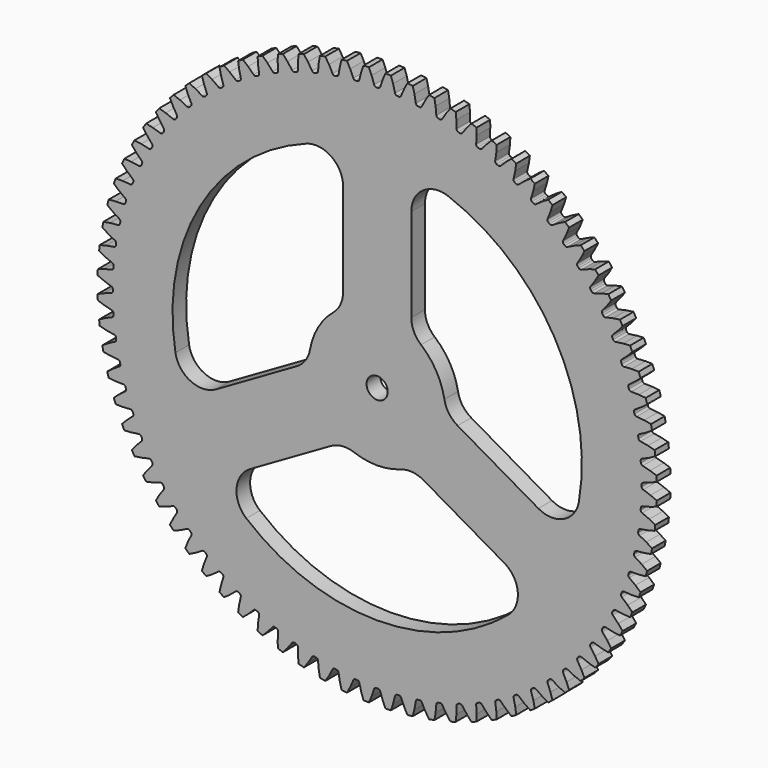
from build123d import *

# Parameters (mm, degrees)
F0_R     = 3.1
F1_DEPTH = 5


# Not quite as in the source:
# - ends of sketch curves that miss each other by under 0.0002 mm in the source are joined


with BuildPart() as f1:
    # F0 (on Front) → F1 (new body)
    with BuildSketch(Plane.XZ):
        with BuildLine():
            ThreePointArc((-66.025163696, 41.5067142777), (-65.8531282029, 41.1183062198), (-65.9498350759, 40.7046580468))
            ThreePointArc((-65.9498350759, 40.7046580468), (-66.0796127847, 40.4936386884), (-66.2087146573, 40.2822057915))
            ThreePointArc((-66.2087146573, 40.2822057915), (-66.5333738388, 40.0082469182), (-66.9575511036, 39.9851986244))
            Line((-66.9575511036, 39.9851986244), (-69.17445, 40.481426))
            Line((-69.17445, 40.481426), (-71.152959, 40.758514))
            ThreePointArc((-71.152959, 40.758514), (-71.5446727033, 40.0669415825), (-71.929665068, 39.3716050372))
            Line((-71.929665068, 39.3716050372), (-70.65964, 37.829428))
            Line((-70.65964, 37.829428), (-69.07821, 36.198488))
            ThreePointArc((-69.07821, 36.198488), (-68.8762309064, 35.8247752552), (-68.9401849616, 35.4048149803))
            ThreePointArc((-68.9401849616, 35.4048149803), (-69.0530056484, 35.1842636831), (-69.1651209082, 34.9633529536))
            ThreePointArc((-69.1651209082, 34.9633529536), (-69.467284766, 34.6647666816), (-69.888344948, 34.6085082698))
            Line((-69.888344948, 34.6085082698), (-72.137344, 34.92927))
            Line((-72.137344, 34.92927), (-74.131494, 35.050273))
            ThreePointArc((-74.131494, 35.050273), (-74.4677401642, 34.3300986722), (-74.7969903852, 33.6066991731))
            Line((-74.7969903852, 33.6066991731), (-73.409883, 32.168921))
            Line((-73.409883, 32.168921), (-71.705366, 30.667087))
            ThreePointArc((-71.705366, 30.667087), (-71.4746875004, 30.3103731451), (-71.5054948793, 29.8866889496))
            ThreePointArc((-71.5054948793, 29.8866889496), (-71.6006637701, 29.6579660072), (-71.695100899, 29.4289399585))
            ThreePointArc((-71.695100899, 29.4289399585), (-71.9729063671, 29.1075663054), (-72.3882550299, 29.0184457338))
            Line((-72.3882550299, 29.0184457338), (-74.655488, 29.161764))
            Line((-74.655488, 29.161764), (-76.652984, 29.125934))
            ThreePointArc((-76.652984, 29.125934), (-76.9316895099, 28.3815987773), (-77.203167309, 27.6345971106))
            Line((-77.203167309, 27.6345971106), (-75.707529, 26.310081))
            Line((-75.707529, 26.310081), (-73.890434, 24.946612))
            ThreePointArc((-73.890434, 24.946612), (-73.6324790283, 24.6090973171), (-73.6299495486, 24.1843018517))
            ThreePointArc((-73.6299495486, 24.1843018517), (-73.7068799327, 23.9488173109), (-73.7830567374, 23.7130879156))
            ThreePointArc((-73.7830567374, 23.7130879156), (-74.0347910448, 23.3709082224), (-74.4418670003, 23.2494739916))
            Line((-74.4418670003, 23.2494739916), (-76.713356, 23.214466))
            Line((-76.713356, 23.214466), (-78.701883, 23.022025))
            ThreePointArc((-78.701883, 23.022025), (-78.9213293367, 22.2581170751), (-79.1333612396, 21.4921180651))
            Line((-79.1333612396, 21.4921180651), (-77.538413, 20.289032))
            Line((-77.538413, 20.289032), (-75.619943, 19.072333))
            ThreePointArc((-75.619943, 19.072333), (-75.3363026573, 18.7560970153), (-75.300452163, 18.3328100397))
            ThreePointArc((-75.300452163, 18.3328100397), (-75.3586689009, 18.092015407), (-75.4161157564, 17.8510359423))
            ThreePointArc((-75.4161157564, 17.8510359423), (-75.640226983, 17.4901601634), (-76.0365209903, 17.3371617849))
            Line((-76.0365209903, 17.3371617849), (-78.29826, 17.124043))
            Line((-78.29826, 17.124043), (-80.265558, 16.776177))
            ThreePointArc((-80.265558, 16.776177), (-80.4243929961, 15.99740639), (-80.5756716705, 15.2171329378))
            Line((-80.5756716705, 15.2171329378), (-78.891247, 14.142894))
            Line((-78.891247, 14.142894), (-76.88323, 13.080467))
            ThreePointArc((-76.88323, 13.080467), (-76.5756525366, 12.7874601089), (-76.5067014576, 12.368291074))
            ThreePointArc((-76.5067014576, 12.368291074), (-76.5458464162, 12.123670914), (-76.5842091605, 11.8789270249))
            ThreePointArc((-76.5842091605, 11.8789270249), (-76.7793160154, 11.5015804485), (-77.1623840176, 11.3179611415))
            Line((-77.1623840176, 11.3179611415), (-79.400429, 10.928045))
            Line((-79.400429, 10.928045), (-81.33437, 10.426899))
            ThreePointArc((-81.33437, 10.426899), (-81.431613449, 9.6380667714), (-81.5212062801, 8.8483290304))
            Line((-81.5212062801, 8.8483290304), (-79.757691, 7.90956))
            Line((-79.757691, 7.90956), (-77.672506, 7.007956))
            ThreePointArc((-77.672506, 7.007956), (-77.3428878657, 6.7399838602), (-77.2412619261, 6.3275169939))
            ThreePointArc((-77.2412619261, 6.3275169939), (-77.2610933521, 6.0805800746), (-77.2801354317, 5.8335810326))
            ThreePointArc((-77.2801354317, 5.8335810326), (-77.4450345987, 5.4420896099), (-77.8125149825, 5.2289809145))
            Line((-77.8125149825, 5.2289809145), (-80.013069, 4.664671))
            Line((-80.013069, 4.664671), (-81.901729, 4.013335))
            ThreePointArc((-81.901729, 4.013335), (-81.936780979, 3.2193047074), (-81.9641355159, 2.4249719857))
            Line((-81.9641355159, 2.4249719857), (-80.132401, 1.627461))
            Line((-80.132401, 1.627461), (-77.982906, 0.892238))
            ThreePointArc((-77.982906, 0.892238), (-77.6332781496, 0.6509548629), (-77.4996034155, 0.2477320013))
            ThreePointArc((-77.4996034155, 0.2477320013), (-77.5, 0), (-77.4996040561, -0.2477320002))
            ThreePointArc((-77.4996040561, -0.2477320002), (-77.6332781496, -0.6509548629), (-77.9829060595, -0.8922387938))
            Line((-77.9829060595, -0.8922387938), (-80.132401, -1.627461))
            Line((-80.132401, -1.627461), (-81.964136, -2.424972))
            ThreePointArc((-81.964136, -2.424972), (-81.936780979, -3.2193047074), (-81.9017285675, -4.0133349788))
            Line((-81.9017285675, -4.0133349788), (-80.013069, -4.664671))
            Line((-80.013069, -4.664671), (-77.812515, -5.228981))
            ThreePointArc((-77.812515, -5.228981), (-77.4450345987, -5.4420896099), (-77.2801356593, -5.8335809743))
            ThreePointArc((-77.2801356593, -5.8335809743), (-77.2610933521, -6.0805800746), (-77.2412618281, -6.3275169859))
            ThreePointArc((-77.2412618281, -6.3275169859), (-77.3428878657, -6.7399838602), (-77.6725058682, -7.0079553509))
            Line((-77.6725058682, -7.0079553509), (-79.757691, -7.90956))
            Line((-79.757691, -7.90956), (-81.521206, -8.848329))
            ThreePointArc((-81.521206, -8.848329), (-81.431613449, -9.6380667714), (-81.3343702053, -10.4268990263))
            Line((-81.3343702053, -10.4268990263), (-79.400429, -10.928045))
            Line((-79.400429, -10.928045), (-77.162384, -11.317961))
            ThreePointArc((-77.162384, -11.317961), (-76.7793160154, -11.5015804485), (-76.5842090848, -11.8789270132))
            ThreePointArc((-76.5842090848, -11.8789270132), (-76.5458464162, -12.123670914), (-76.5067015339, -12.3682909247))
            ThreePointArc((-76.5067015339, -12.3682909247), (-76.5756525366, -12.7874601089), (-76.8832300047, -13.0804669899))
            Line((-76.8832300047, -13.0804669899), (-78.891247, -14.142894))
            Line((-78.891247, -14.142894), (-80.575672, -15.217133))
            ThreePointArc((-80.575672, -15.217133), (-80.4243929961, -15.99740639), (-80.2655585445, -16.7761769048))
            Line((-80.2655585445, -16.7761769048), (-78.29826, -17.124043))
            Line((-78.29826, -17.124043), (-76.036521, -17.337162))
            ThreePointArc((-76.036521, -17.337162), (-75.640226983, -17.4901601634), (-75.4161153834, -17.8510360908))
            ThreePointArc((-75.4161153834, -17.8510360908), (-75.3586689009, -18.092015407), (-75.3004520382, -18.3328100093))
            ThreePointArc((-75.3004520382, -18.3328100093), (-75.3363026573, -18.7560970153), (-75.6199428543, -19.0723332566))
            Line((-75.6199428543, -19.0723332566), (-77.538413, -20.289032))
            Line((-77.538413, -20.289032), (-79.133361, -21.492118))
            ThreePointArc((-79.133361, -21.492118), (-78.9213293367, -22.2581170751), (-78.7018828663, -23.0220249609))
            Line((-78.7018828663, -23.0220249609), (-76.713356, -23.214466))
            Line((-76.713356, -23.214466), (-74.441867, -23.249474))
            ThreePointArc((-74.441867, -23.249474), (-74.0347910448, -23.3709082224), (-73.7830567306, -23.7130879134))
            ThreePointArc((-73.7830567306, -23.7130879134), (-73.7068799327, -23.9488173109), (-73.6299499986, -24.1843019995))
            ThreePointArc((-73.6299499986, -24.1843019995), (-73.6324790283, -24.6090973171), (-73.8904340374, -24.9466129447))
            Line((-73.8904340374, -24.9466129447), (-75.707529, -26.310081))
            Line((-75.707529, -26.310081), (-77.203168, -27.634597))
            ThreePointArc((-77.203168, -27.634597), (-76.9316895099, -28.3815987773), (-76.6529840714, -29.1259340271))
            Line((-76.6529840714, -29.1259340271), (-74.655488, -29.161764))
            Line((-74.655488, -29.161764), (-72.388255, -29.018446))
            ThreePointArc((-72.388255, -29.018446), (-71.9729063671, -29.1075663054), (-71.6951006076, -29.4289398389))
            ThreePointArc((-71.6951006076, -29.4289398389), (-71.6006637701, -29.6579660072), (-71.5054950323, -29.8866890135))
            ThreePointArc((-71.5054950323, -29.8866890135), (-71.4746875004, -30.3103731451), (-71.7053658896, -30.6670871383))
            Line((-71.7053658896, -30.6670871383), (-73.409883, -32.168921))
            Line((-73.409883, -32.168921), (-74.79699, -33.606699))
            ThreePointArc((-74.79699, -33.606699), (-74.4677401642, -34.3300986722), (-74.1314937792, -35.0502728956))
            Line((-74.1314937792, -35.0502728956), (-72.137344, -34.92927))
            Line((-72.137344, -34.92927), (-69.888345, -34.608508))
            ThreePointArc((-69.888345, -34.608508), (-69.467284766, -34.6647666816), (-69.16512115, -34.9633530758))
            ThreePointArc((-69.16512115, -34.9633530758), (-69.0530056484, -35.1842636831), (-68.9401848105, -35.4048149027))
            ThreePointArc((-68.9401848105, -35.4048149027), (-68.8762309064, -35.8247752552), (-69.0782100408, -36.1984879563))
            Line((-69.0782100408, -36.1984879563), (-70.65964, -37.829428))
            Line((-70.65964, -37.829428), (-71.929665, -39.371605))
            ThreePointArc((-71.929665, -39.371605), (-71.5446727033, -40.0669415825), (-71.1529587992, -40.758513885))
            Line((-71.1529587992, -40.758513885), (-69.17445, -40.481426))
            Line((-69.17445, -40.481426), (-66.957551, -39.985198))
            ThreePointArc((-66.957551, -39.985198), (-66.5333738388, -40.0082469182), (-66.208714043, -40.2822060261))
            ThreePointArc((-66.208714043, -40.2822060261), (-66.0796127847, -40.4936386884), (-65.9498357182, -40.7046578261))
            ThreePointArc((-65.9498357182, -40.7046578261), (-65.8531282029, -41.1183062198), (-66.025163696, -41.5067142777))
            Line((-66.025163696, -41.5067142777), (-67.473758, -43.256704))
            Line((-67.473758, -43.256704), (-68.618869, -44.893772))
            ThreePointArc((-68.618869, -44.893772), (-68.1805082686, -45.5567590182), (-67.735741789, -46.215465856))
            Line((-67.735741789, -46.215465856), (-65.785072, -45.784))
            Line((-65.785072, -45.784), (-63.61394, -45.115366))
            ThreePointArc((-63.61394, -45.115366), (-63.1892626446, -45.1050629786), (-62.8441095983, -45.3527047101))
            ThreePointArc((-62.8441095983, -45.3527047101), (-62.6988173077, -45.5533567174), (-62.5528840324, -45.7535430237))
            ThreePointArc((-62.5528840324, -45.7535430237), (-62.4240202675, -46.1583290518), (-62.5650518603, -46.5590381088))
            Line((-62.5650518603, -46.5590381088), (-63.871877, -48.417288))
            Line((-63.871877, -48.417288), (-64.885016, -50.139154))
            ThreePointArc((-64.885016, -50.139154), (-64.3959884553, -50.7657036873), (-63.9009112923, -51.3874842351))
            Line((-63.9009112923, -51.3874842351), (-61.990108, -50.8043))
            Line((-61.990108, -50.8043), (-59.878129, -49.967383))
            ThreePointArc((-59.878129, -49.967383), (-59.4555689615, -49.9237918029), (-59.0920500504, -50.1435900427))
            ThreePointArc((-59.0920500504, -50.1435900427), (-58.9314622753, -50.3322238143), (-58.7702723533, -50.5203433037))
            ThreePointArc((-58.7702723533, -50.5203433037), (-58.6100466547, -50.9137703875), (-58.7192039287, -51.324309047))
            Line((-58.7192039287, -51.324309047), (-59.876204, -53.279363))
            Line((-59.876204, -53.279363), (-60.751124, -55.075411))
            ThreePointArc((-60.751124, -55.075411), (-60.2144456457, -55.6616612722), (-59.6721100426, -56.2426820401))
            Line((-59.6721100426, -56.2426820401), (-57.812953, -55.511375))
            Line((-57.812953, -55.511375), (-55.773149, -54.511334))
            ThreePointArc((-55.773149, -54.511334), (-55.3553116325, -54.4347236217), (-54.9756682141, -54.6253232127))
            ThreePointArc((-54.9756682141, -54.6253232127), (-54.800775542, -54.800775542), (-54.6253230687, -54.9756680691))
            ThreePointArc((-54.6253230687, -54.9756680691), (-54.4347236217, -55.3553116325), (-54.5113336317, -55.7731492035))
            Line((-54.5113336317, -55.7731492035), (-55.511375, -57.812953))
            Line((-55.511375, -57.812953), (-56.242682, -59.67211))
            ThreePointArc((-56.242682, -59.67211), (-55.6616612722, -60.2144456457), (-55.0754111471, -60.7511241623))
            Line((-55.0754111471, -60.7511241623), (-53.279363, -59.876204))
            Line((-53.279363, -59.876204), (-51.324309, -58.719204))
            ThreePointArc((-51.324309, -58.719204), (-50.9137703875, -58.6100466547), (-50.5203429251, -58.7702719129))
            ThreePointArc((-50.5203429251, -58.7702719129), (-50.3322238143, -58.9314622753), (-50.1435900364, -59.0920500428))
            ThreePointArc((-50.1435900364, -59.0920500428), (-49.9237918029, -59.4555689615), (-49.9673827084, -59.8781291324))
            Line((-49.9673827084, -59.8781291324), (-50.8043, -61.990108))
            Line((-50.8043, -61.990108), (-51.387484, -63.900911))
            ThreePointArc((-51.387484, -63.900911), (-50.7657036873, -64.3959884553), (-50.1391537571, -64.8850156856))
            Line((-50.1391537571, -64.8850156856), (-48.417288, -63.871877))
            Line((-48.417288, -63.871877), (-46.559038, -62.565052))
            ThreePointArc((-46.559038, -62.565052), (-46.1583290518, -62.4240202675), (-45.7535428924, -62.5528838529))
            ThreePointArc((-45.7535428924, -62.5528838529), (-45.5533567174, -62.6988173077), (-45.3527049528, -62.8441099346))
            ThreePointArc((-45.3527049528, -62.8441099346), (-45.1050629786, -63.1892626446), (-45.1153658461, -63.6139400558))
            Line((-45.1153658461, -63.6139400558), (-45.784, -65.785072))
            Line((-45.784, -65.785072), (-46.215466, -67.735742))
            ThreePointArc((-46.215466, -67.735742), (-45.5567590182, -68.1805082686), (-44.8937721762, -68.6188692693))
            Line((-44.8937721762, -68.6188692693), (-43.256704, -67.473758))
            Line((-43.256704, -67.473758), (-41.506714, -66.025164))
            ThreePointArc((-41.506714, -66.025164), (-41.1183062198, -65.8531282029), (-40.7046580468, -65.9498350759))
            ThreePointArc((-40.7046580468, -65.9498350759), (-40.4936386884, -66.0796127847), (-40.2822057915, -66.2087146573))
            ThreePointArc((-40.2822057915, -66.2087146573), (-40.0082469182, -66.5333738388), (-39.9851986244, -66.9575511036))
            Line((-39.9851986244, -66.9575511036), (-40.481426, -69.17445))
            Line((-40.481426, -69.17445), (-40.758514, -71.152959))
            ThreePointArc((-40.758514, -71.152959), (-40.0669415825, -71.5446727033), (-39.3716050372, -71.929665068))
            Line((-39.3716050372, -71.929665068), (-37.829428, -70.65964))
            Line((-37.829428, -70.65964), (-36.198488, -69.07821))
            ThreePointArc((-36.198488, -69.07821), (-35.8247752552, -68.8762309064), (-35.4048149803, -68.9401849616))
            ThreePointArc((-35.4048149803, -68.9401849616), (-35.1842636831, -69.0530056484), (-34.9633529536, -69.1651209082))
            ThreePointArc((-34.9633529536, -69.1651209082), (-34.6647666816, -69.467284766), (-34.6085082698, -69.888344948))
            Line((-34.6085082698, -69.888344948), (-34.92927, -72.137344))
            Line((-34.92927, -72.137344), (-35.050273, -74.131494))
            ThreePointArc((-35.050273, -74.131494), (-34.3300986722, -74.4677401642), (-33.6066991731, -74.7969903852))
            Line((-33.6066991731, -74.7969903852), (-32.168921, -73.409883))
            Line((-32.168921, -73.409883), (-30.667087, -71.705366))
            ThreePointArc((-30.667087, -71.705366), (-30.3103731451, -71.4746875004), (-29.8866889496, -71.5054948793))
            ThreePointArc((-29.8866889496, -71.5054948793), (-29.6579660072, -71.6006637701), (-29.4289399585, -71.695100899))
            ThreePointArc((-29.4289399585, -71.695100899), (-29.1075663054, -71.9729063671), (-29.0184457338, -72.3882550299))
            Line((-29.0184457338, -72.3882550299), (-29.161764, -74.655488))
            Line((-29.161764, -74.655488), (-29.125934, -76.652984))
            ThreePointArc((-29.125934, -76.652984), (-28.3815987773, -76.9316895099), (-27.6345971106, -77.203167309))
            Line((-27.6345971106, -77.203167309), (-26.310081, -75.707529))
            Line((-26.310081, -75.707529), (-24.946612, -73.890434))
            ThreePointArc((-24.946612, -73.890434), (-24.6090973171, -73.6324790283), (-24.1843018517, -73.6299495486))
            ThreePointArc((-24.1843018517, -73.6299495486), (-23.9488173109, -73.7068799327), (-23.7130879156, -73.7830567374))
            ThreePointArc((-23.7130879156, -73.7830567374), (-23.3709082224, -74.0347910448), (-23.2494739916, -74.4418670003))
            Line((-23.2494739916, -74.4418670003), (-23.214466, -76.713356))
            Line((-23.214466, -76.713356), (-23.022025, -78.701883))
            ThreePointArc((-23.022025, -78.701883), (-22.2581170751, -78.9213293367), (-21.4921180651, -79.1333612396))
            Line((-21.4921180651, -79.1333612396), (-20.289032, -77.538413))
            Line((-20.289032, -77.538413), (-19.072333, -75.619943))
            ThreePointArc((-19.072333, -75.619943), (-18.7560970153, -75.3363026573), (-18.3328100397, -75.300452163))
            ThreePointArc((-18.3328100397, -75.300452163), (-18.092015407, -75.3586689009), (-17.8510359423, -75.4161157564))
            ThreePointArc((-17.8510359423, -75.4161157564), (-17.4901601634, -75.640226983), (-17.3371617849, -76.0365209903))
            Line((-17.3371617849, -76.0365209903), (-17.124043, -78.29826))
            Line((-17.124043, -78.29826), (-16.776177, -80.265558))
            ThreePointArc((-16.776177, -80.265558), (-15.99740639, -80.4243929961), (-15.2171329378, -80.5756716705))
            Line((-15.2171329378, -80.5756716705), (-14.142894, -78.891247))
            Line((-14.142894, -78.891247), (-13.080467, -76.88323))
            ThreePointArc((-13.080467, -76.88323), (-12.7874601089, -76.5756525366), (-12.368291074, -76.5067014576))
            ThreePointArc((-12.368291074, -76.5067014576), (-12.123670914, -76.5458464162), (-11.8789270249, -76.5842091605))
            ThreePointArc((-11.8789270249, -76.5842091605), (-11.5015804485, -76.7793160154), (-11.3179611415, -77.1623840176))
            Line((-11.3179611415, -77.1623840176), (-10.928045, -79.400429))
            Line((-10.928045, -79.400429), (-10.426899, -81.33437))
            ThreePointArc((-10.426899, -81.33437), (-9.6380667714, -81.431613449), (-8.8483290304, -81.5212062801))
            Line((-8.8483290304, -81.5212062801), (-7.90956, -79.757691))
            Line((-7.90956, -79.757691), (-7.007956, -77.672506))
            ThreePointArc((-7.007956, -77.672506), (-6.7399838602, -77.3428878657), (-6.3275169939, -77.2412619261))
            ThreePointArc((-6.3275169939, -77.2412619261), (-6.0805800746, -77.2610933521), (-5.8335810326, -77.2801354317))
            ThreePointArc((-5.8335810326, -77.2801354317), (-5.4420896099, -77.4450345987), (-5.2289809145, -77.8125149825))
            Line((-5.2289809145, -77.8125149825), (-4.664671, -80.013069))
            Line((-4.664671, -80.013069), (-4.013335, -81.901729))
            ThreePointArc((-4.013335, -81.901729), (-3.2193047074, -81.936780979), (-2.4249719857, -81.9641355159))
            Line((-2.4249719857, -81.9641355159), (-1.627461, -80.132401))
            Line((-1.627461, -80.132401), (-0.892238, -77.982906))
            ThreePointArc((-0.892238, -77.982906), (-0.6509548629, -77.6332781496), (-0.2477320013, -77.4996034155))
            ThreePointArc((-0.2477320013, -77.4996034155), (0, -77.5), (0.2477320002, -77.4996040561))
            ThreePointArc((0.2477320002, -77.4996040561), (0.6509548629, -77.6332781496), (0.8922387938, -77.9829060595))
            Line((0.8922387938, -77.9829060595), (1.627461, -80.132401))
            Line((1.627461, -80.132401), (2.424972, -81.964136))
            ThreePointArc((2.424972, -81.964136), (3.2193047074, -81.936780979), (4.0133349788, -81.9017285675))
            Line((4.0133349788, -81.9017285675), (4.664671, -80.013069))
            Line((4.664671, -80.013069), (5.228981, -77.812515))
            ThreePointArc((5.228981, -77.812515), (5.4420896099, -77.4450345987), (5.8335809743, -77.2801356593))
            ThreePointArc((5.8335809743, -77.2801356593), (6.0805800746, -77.2610933521), (6.3275169859, -77.2412618281))
            ThreePointArc((6.3275169859, -77.2412618281), (6.7399838602, -77.3428878657), (7.0079553509, -77.6725058682))
            Line((7.0079553509, -77.6725058682), (7.90956, -79.757691))
            Line((7.90956, -79.757691), (8.848329, -81.521206))
            ThreePointArc((8.848329, -81.521206), (9.6380667714, -81.431613449), (10.4268990263, -81.3343702053))
            Line((10.4268990263, -81.3343702053), (10.928045, -79.400429))
            Line((10.928045, -79.400429), (11.317961, -77.162384))
            ThreePointArc((11.317961, -77.162384), (11.5015804485, -76.7793160154), (11.8789270132, -76.5842090848))
            ThreePointArc((11.8789270132, -76.5842090848), (12.123670914, -76.5458464162), (12.3682909247, -76.5067015339))
            ThreePointArc((12.3682909247, -76.5067015339), (12.7874601089, -76.5756525366), (13.0804669899, -76.8832300047))
            Line((13.0804669899, -76.8832300047), (14.142894, -78.891247))
            Line((14.142894, -78.891247), (15.217133, -80.575672))
            ThreePointArc((15.217133, -80.575672), (15.99740639, -80.4243929961), (16.7761769048, -80.2655585445))
            Line((16.7761769048, -80.2655585445), (17.124043, -78.29826))
            Line((17.124043, -78.29826), (17.337162, -76.036521))
            ThreePointArc((17.337162, -76.036521), (17.4901601634, -75.640226983), (17.8510360908, -75.4161153834))
            ThreePointArc((17.8510360908, -75.4161153834), (18.092015407, -75.3586689009), (18.3328100093, -75.3004520382))
            ThreePointArc((18.3328100093, -75.3004520382), (18.7560970153, -75.3363026573), (19.0723332566, -75.6199428543))
            Line((19.0723332566, -75.6199428543), (20.289032, -77.538413))
            Line((20.289032, -77.538413), (21.492118, -79.133361))
            ThreePointArc((21.492118, -79.133361), (22.2581170751, -78.9213293367), (23.0220249609, -78.7018828663))
            Line((23.0220249609, -78.7018828663), (23.214466, -76.713356))
            Line((23.214466, -76.713356), (23.249474, -74.441867))
            ThreePointArc((23.249474, -74.441867), (23.3709082224, -74.0347910448), (23.7130879134, -73.7830567306))
            ThreePointArc((23.7130879134, -73.7830567306), (23.9488173109, -73.7068799327), (24.1843019995, -73.6299499986))
            ThreePointArc((24.1843019995, -73.6299499986), (24.6090973171, -73.6324790283), (24.9466129447, -73.8904340374))
            Line((24.9466129447, -73.8904340374), (26.310081, -75.707529))
            Line((26.310081, -75.707529), (27.634597, -77.203168))
            ThreePointArc((27.634597, -77.203168), (28.3815987773, -76.9316895099), (29.1259340271, -76.6529840714))
            Line((29.1259340271, -76.6529840714), (29.161764, -74.655488))
            Line((29.161764, -74.655488), (29.018446, -72.388255))
            ThreePointArc((29.018446, -72.388255), (29.1075663054, -71.9729063671), (29.4289398389, -71.6951006076))
            ThreePointArc((29.4289398389, -71.6951006076), (29.6579660072, -71.6006637701), (29.8866890135, -71.5054950323))
            ThreePointArc((29.8866890135, -71.5054950323), (30.3103731451, -71.4746875004), (30.6670871383, -71.7053658896))
            Line((30.6670871383, -71.7053658896), (32.168921, -73.409883))
            Line((32.168921, -73.409883), (33.606699, -74.79699))
            ThreePointArc((33.606699, -74.79699), (34.3300986722, -74.4677401642), (35.0502728956, -74.1314937792))
            Line((35.0502728956, -74.1314937792), (34.92927, -72.137344))
            Line((34.92927, -72.137344), (34.608508, -69.888345))
            ThreePointArc((34.608508, -69.888345), (34.6647666816, -69.467284766), (34.9633530758, -69.16512115))
            ThreePointArc((34.9633530758, -69.16512115), (35.1842636831, -69.0530056484), (35.4048149027, -68.9401848105))
            ThreePointArc((35.4048149027, -68.9401848105), (35.8247752552, -68.8762309064), (36.1984879563, -69.0782100408))
            Line((36.1984879563, -69.0782100408), (37.829428, -70.65964))
            Line((37.829428, -70.65964), (39.371605, -71.929665))
            ThreePointArc((39.371605, -71.929665), (40.0669415825, -71.5446727033), (40.758513885, -71.1529587992))
            Line((40.758513885, -71.1529587992), (40.481426, -69.17445))
            Line((40.481426, -69.17445), (39.985198, -66.957551))
            ThreePointArc((39.985198, -66.957551), (40.0082469182, -66.5333738388), (40.2822060261, -66.208714043))
            ThreePointArc((40.2822060261, -66.208714043), (40.4936386884, -66.0796127847), (40.7046578261, -65.9498357182))
            ThreePointArc((40.7046578261, -65.9498357182), (41.1183062198, -65.8531282029), (41.5067142777, -66.025163696))
            Line((41.5067142777, -66.025163696), (43.256704, -67.473758))
            Line((43.256704, -67.473758), (44.893772, -68.618869))
            ThreePointArc((44.893772, -68.618869), (45.5567590182, -68.1805082686), (46.215465856, -67.735741789))
            Line((46.215465856, -67.735741789), (45.784, -65.785072))
            Line((45.784, -65.785072), (45.115366, -63.61394))
            ThreePointArc((45.115366, -63.61394), (45.1050629786, -63.1892626446), (45.3527047101, -62.8441095983))
            ThreePointArc((45.3527047101, -62.8441095983), (45.5533567174, -62.6988173077), (45.7535430237, -62.5528840324))
            ThreePointArc((45.7535430237, -62.5528840324), (46.1583290518, -62.4240202675), (46.5590381088, -62.5650518603))
            Line((46.5590381088, -62.5650518603), (48.417288, -63.871877))
            Line((48.417288, -63.871877), (50.139154, -64.885016))
            ThreePointArc((50.139154, -64.885016), (50.7657036873, -64.3959884553), (51.3874842351, -63.9009112923))
            Line((51.3874842351, -63.9009112923), (50.8043, -61.990108))
            Line((50.8043, -61.990108), (49.967383, -59.878129))
            ThreePointArc((49.967383, -59.878129), (49.9237918029, -59.4555689615), (50.1435900427, -59.0920500504))
            ThreePointArc((50.1435900427, -59.0920500504), (50.3322238143, -58.9314622753), (50.5203433037, -58.7702723533))
            ThreePointArc((50.5203433037, -58.7702723533), (50.9137703875, -58.6100466547), (51.324309047, -58.7192039287))
            Line((51.324309047, -58.7192039287), (53.279363, -59.876204))
            Line((53.279363, -59.876204), (55.075411, -60.751124))
            ThreePointArc((55.075411, -60.751124), (55.6616612722, -60.2144456457), (56.2426820401, -59.6721100426))
            Line((56.2426820401, -59.6721100426), (55.511375, -57.812953))
            Line((55.511375, -57.812953), (54.511334, -55.773149))
            ThreePointArc((54.511334, -55.773149), (54.4347236217, -55.3553116325), (54.6253232127, -54.9756682141))
            ThreePointArc((54.6253232127, -54.9756682141), (54.800775542, -54.800775542), (54.9756680691, -54.6253230687))
            ThreePointArc((54.9756680691, -54.6253230687), (55.3553116325, -54.4347236217), (55.7731492035, -54.5113336317))
            Line((55.7731492035, -54.5113336317), (57.812953, -55.511375))
            Line((57.812953, -55.511375), (59.67211, -56.242682))
            ThreePointArc((59.67211, -56.242682), (60.2144456457, -55.6616612722), (60.7511241623, -55.0754111471))
            Line((60.7511241623, -55.0754111471), (59.876204, -53.279363))
            Line((59.876204, -53.279363), (58.719204, -51.324309))
            ThreePointArc((58.719204, -51.324309), (58.6100466547, -50.9137703875), (58.7702719129, -50.5203429251))
            ThreePointArc((58.7702719129, -50.5203429251), (58.9314622753, -50.3322238143), (59.0920500428, -50.1435900364))
            ThreePointArc((59.0920500428, -50.1435900364), (59.4555689615, -49.9237918029), (59.8781291324, -49.9673827084))
            Line((59.8781291324, -49.9673827084), (61.990108, -50.8043))
            Line((61.990108, -50.8043), (63.900911, -51.387484))
            ThreePointArc((63.900911, -51.387484), (64.3959884553, -50.7657036873), (64.8850156856, -50.1391537571))
            Line((64.8850156856, -50.1391537571), (63.871877, -48.417288))
            Line((63.871877, -48.417288), (62.565052, -46.559038))
            ThreePointArc((62.565052, -46.559038), (62.4240202675, -46.1583290518), (62.5528838529, -45.7535428924))
            ThreePointArc((62.5528838529, -45.7535428924), (62.6988173077, -45.5533567174), (62.8441099346, -45.3527049528))
            ThreePointArc((62.8441099346, -45.3527049528), (63.1892626446, -45.1050629786), (63.6139400558, -45.1153658461))
            Line((63.6139400558, -45.1153658461), (65.785072, -45.784))
            Line((65.785072, -45.784), (67.735742, -46.215466))
            ThreePointArc((67.735742, -46.215466), (68.1805082686, -45.5567590182), (68.6188692693, -44.8937721762))
            Line((68.6188692693, -44.8937721762), (67.473758, -43.256704))
            Line((67.473758, -43.256704), (66.025164, -41.506714))
            ThreePointArc((66.025164, -41.506714), (65.8531282029, -41.1183062198), (65.9498350759, -40.7046580468))
            ThreePointArc((65.9498350759, -40.7046580468), (66.0796127847, -40.4936386884), (66.2087146573, -40.2822057915))
            ThreePointArc((66.2087146573, -40.2822057915), (66.5333738388, -40.0082469182), (66.9575511036, -39.9851986244))
            Line((66.9575511036, -39.9851986244), (69.17445, -40.481426))
            Line((69.17445, -40.481426), (71.152959, -40.758514))
            ThreePointArc((71.152959, -40.758514), (71.5446727033, -40.0669415825), (71.929665068, -39.3716050372))
            Line((71.929665068, -39.3716050372), (70.65964, -37.829428))
            Line((70.65964, -37.829428), (69.07821, -36.198488))
            ThreePointArc((69.07821, -36.198488), (68.8762309064, -35.8247752552), (68.9401849616, -35.4048149803))
            ThreePointArc((68.9401849616, -35.4048149803), (69.0530056484, -35.1842636831), (69.1651209082, -34.9633529536))
            ThreePointArc((69.1651209082, -34.9633529536), (69.467284766, -34.6647666816), (69.888344948, -34.6085082698))
            Line((69.888344948, -34.6085082698), (72.137344, -34.92927))
            Line((72.137344, -34.92927), (74.131494, -35.050273))
            ThreePointArc((74.131494, -35.050273), (74.4677401642, -34.3300986722), (74.7969903852, -33.6066991731))
            Line((74.7969903852, -33.6066991731), (73.409883, -32.168921))
            Line((73.409883, -32.168921), (71.705366, -30.667087))
            ThreePointArc((71.705366, -30.667087), (71.4746875004, -30.3103731451), (71.5054948793, -29.8866889496))
            ThreePointArc((71.5054948793, -29.8866889496), (71.6006637701, -29.6579660072), (71.695100899, -29.4289399585))
            ThreePointArc((71.695100899, -29.4289399585), (71.9729063671, -29.1075663054), (72.3882550299, -29.0184457338))
            Line((72.3882550299, -29.0184457338), (74.655488, -29.161764))
            Line((74.655488, -29.161764), (76.652984, -29.125934))
            ThreePointArc((76.652984, -29.125934), (76.9316895099, -28.3815987773), (77.203167309, -27.6345971106))
            Line((77.203167309, -27.6345971106), (75.707529, -26.310081))
            Line((75.707529, -26.310081), (73.890434, -24.946612))
            ThreePointArc((73.890434, -24.946612), (73.6324790283, -24.6090973171), (73.6299495486, -24.1843018517))
            ThreePointArc((73.6299495486, -24.1843018517), (73.7068799327, -23.9488173109), (73.7830567374, -23.7130879156))
            ThreePointArc((73.7830567374, -23.7130879156), (74.0347910448, -23.3709082224), (74.4418670003, -23.2494739916))
            Line((74.4418670003, -23.2494739916), (76.713356, -23.214466))
            Line((76.713356, -23.214466), (78.701883, -23.022025))
            ThreePointArc((78.701883, -23.022025), (78.9213293367, -22.2581170751), (79.1333612396, -21.4921180651))
            Line((79.1333612396, -21.4921180651), (77.538413, -20.289032))
            Line((77.538413, -20.289032), (75.619943, -19.072333))
            ThreePointArc((75.619943, -19.072333), (75.3363026573, -18.7560970153), (75.300452163, -18.3328100397))
            ThreePointArc((75.300452163, -18.3328100397), (75.3586689009, -18.092015407), (75.4161157564, -17.8510359423))
            ThreePointArc((75.4161157564, -17.8510359423), (75.640226983, -17.4901601634), (76.0365209903, -17.3371617849))
            Line((76.0365209903, -17.3371617849), (78.29826, -17.124043))
            Line((78.29826, -17.124043), (80.265558, -16.776177))
            ThreePointArc((80.265558, -16.776177), (80.4243929961, -15.99740639), (80.5756716705, -15.2171329378))
            Line((80.5756716705, -15.2171329378), (78.891247, -14.142894))
            Line((78.891247, -14.142894), (76.88323, -13.080467))
            ThreePointArc((76.88323, -13.080467), (76.5756525366, -12.7874601089), (76.5067014576, -12.368291074))
            ThreePointArc((76.5067014576, -12.368291074), (76.5458464162, -12.123670914), (76.5842091605, -11.8789270249))
            ThreePointArc((76.5842091605, -11.8789270249), (76.7793160154, -11.5015804485), (77.1623840176, -11.3179611415))
            Line((77.1623840176, -11.3179611415), (79.400429, -10.928045))
            Line((79.400429, -10.928045), (81.33437, -10.426899))
            ThreePointArc((81.33437, -10.426899), (81.431613449, -9.6380667714), (81.5212062801, -8.8483290304))
            Line((81.5212062801, -8.8483290304), (79.757691, -7.90956))
            Line((79.757691, -7.90956), (77.672506, -7.007956))
            ThreePointArc((77.672506, -7.007956), (77.3428878657, -6.7399838602), (77.2412619261, -6.3275169939))
            ThreePointArc((77.2412619261, -6.3275169939), (77.2610933521, -6.0805800746), (77.2801354317, -5.8335810326))
            ThreePointArc((77.2801354317, -5.8335810326), (77.4450345987, -5.4420896099), (77.8125149825, -5.2289809145))
            Line((77.8125149825, -5.2289809145), (80.013069, -4.664671))
            Line((80.013069, -4.664671), (81.901729, -4.013335))
            ThreePointArc((81.901729, -4.013335), (81.936780979, -3.2193047074), (81.9641355159, -2.4249719857))
            Line((81.9641355159, -2.4249719857), (80.132401, -1.627461))
            Line((80.132401, -1.627461), (77.982906, -0.892238))
            ThreePointArc((77.982906, -0.892238), (77.6332781496, -0.6509548629), (77.4996034155, -0.2477320013))
            ThreePointArc((77.4996034155, -0.2477320013), (77.5, 0), (77.4996040561, 0.2477320002))
            ThreePointArc((77.4996040561, 0.2477320002), (77.6332781496, 0.6509548629), (77.9829060595, 0.8922387938))
            Line((77.9829060595, 0.8922387938), (80.132401, 1.627461))
            Line((80.132401, 1.627461), (81.964136, 2.424972))
            ThreePointArc((81.964136, 2.424972), (81.936780979, 3.2193047074), (81.9017285675, 4.0133349788))
            Line((81.9017285675, 4.0133349788), (80.013069, 4.664671))
            Line((80.013069, 4.664671), (77.812515, 5.228981))
            ThreePointArc((77.812515, 5.228981), (77.4450345987, 5.4420896099), (77.2801356593, 5.8335809743))
            ThreePointArc((77.2801356593, 5.8335809743), (77.2610933521, 6.0805800746), (77.2412618281, 6.3275169859))
            ThreePointArc((77.2412618281, 6.3275169859), (77.3428878657, 6.7399838602), (77.6725058682, 7.0079553509))
            Line((77.6725058682, 7.0079553509), (79.757691, 7.90956))
            Line((79.757691, 7.90956), (81.521206, 8.848329))
            ThreePointArc((81.521206, 8.848329), (81.431613449, 9.6380667714), (81.3343702053, 10.4268990263))
            Line((81.3343702053, 10.4268990263), (79.400429, 10.928045))
            Line((79.400429, 10.928045), (77.162384, 11.317961))
            ThreePointArc((77.162384, 11.317961), (76.7793160154, 11.5015804485), (76.5842090848, 11.8789270132))
            ThreePointArc((76.5842090848, 11.8789270132), (76.5458464162, 12.123670914), (76.5067015339, 12.3682909247))
            ThreePointArc((76.5067015339, 12.3682909247), (76.5756525366, 12.7874601089), (76.8832300047, 13.0804669899))
            Line((76.8832300047, 13.0804669899), (78.891247, 14.142894))
            Line((78.891247, 14.142894), (80.575672, 15.217133))
            ThreePointArc((80.575672, 15.217133), (80.4243929961, 15.99740639), (80.2655585445, 16.7761769048))
            Line((80.2655585445, 16.7761769048), (78.29826, 17.124043))
            Line((78.29826, 17.124043), (76.036521, 17.337162))
            ThreePointArc((76.036521, 17.337162), (75.640226983, 17.4901601634), (75.4161153834, 17.8510360908))
            ThreePointArc((75.4161153834, 17.8510360908), (75.3586689009, 18.092015407), (75.3004520382, 18.3328100093))
            ThreePointArc((75.3004520382, 18.3328100093), (75.3363026573, 18.7560970153), (75.6199428543, 19.0723332566))
            Line((75.6199428543, 19.0723332566), (77.538413, 20.289032))
            Line((77.538413, 20.289032), (79.133361, 21.492118))
            ThreePointArc((79.133361, 21.492118), (78.9213293367, 22.2581170751), (78.7018828663, 23.0220249609))
            Line((78.7018828663, 23.0220249609), (76.713356, 23.214466))
            Line((76.713356, 23.214466), (74.441867, 23.249474))
            ThreePointArc((74.441867, 23.249474), (74.0347910448, 23.3709082224), (73.7830567306, 23.7130879134))
            ThreePointArc((73.7830567306, 23.7130879134), (73.7068799327, 23.9488173109), (73.6299499986, 24.1843019995))
            ThreePointArc((73.6299499986, 24.1843019995), (73.6324790283, 24.6090973171), (73.8904340374, 24.9466129447))
            Line((73.8904340374, 24.9466129447), (75.707529, 26.310081))
            Line((75.707529, 26.310081), (77.203168, 27.634597))
            ThreePointArc((77.203168, 27.634597), (76.9316895099, 28.3815987773), (76.6529840714, 29.1259340271))
            Line((76.6529840714, 29.1259340271), (74.655488, 29.161764))
            Line((74.655488, 29.161764), (72.388255, 29.018446))
            ThreePointArc((72.388255, 29.018446), (71.9729063671, 29.1075663054), (71.6951006076, 29.4289398389))
            ThreePointArc((71.6951006076, 29.4289398389), (71.6006637701, 29.6579660072), (71.5054950323, 29.8866890135))
            ThreePointArc((71.5054950323, 29.8866890135), (71.4746875004, 30.3103731451), (71.7053658896, 30.6670871383))
            Line((71.7053658896, 30.6670871383), (73.409883, 32.168921))
            Line((73.409883, 32.168921), (74.79699, 33.606699))
            ThreePointArc((74.79699, 33.606699), (74.4677401642, 34.3300986722), (74.1314937792, 35.0502728956))
            Line((74.1314937792, 35.0502728956), (72.137344, 34.92927))
            Line((72.137344, 34.92927), (69.888345, 34.608508))
            ThreePointArc((69.888345, 34.608508), (69.467284766, 34.6647666816), (69.16512115, 34.9633530758))
            ThreePointArc((69.16512115, 34.9633530758), (69.0530056484, 35.1842636831), (68.9401848105, 35.4048149027))
            ThreePointArc((68.9401848105, 35.4048149027), (68.8762309064, 35.8247752552), (69.0782100408, 36.1984879563))
            Line((69.0782100408, 36.1984879563), (70.65964, 37.829428))
            Line((70.65964, 37.829428), (71.929665, 39.371605))
            ThreePointArc((71.929665, 39.371605), (71.5446727033, 40.0669415825), (71.1529587992, 40.758513885))
            Line((71.1529587992, 40.758513885), (69.17445, 40.481426))
            Line((69.17445, 40.481426), (66.957551, 39.985198))
            ThreePointArc((66.957551, 39.985198), (66.5333738388, 40.0082469182), (66.208714043, 40.2822060261))
            ThreePointArc((66.208714043, 40.2822060261), (66.0796127847, 40.4936386884), (65.9498357182, 40.7046578261))
            ThreePointArc((65.9498357182, 40.7046578261), (65.8531282029, 41.1183062198), (66.025163696, 41.5067142777))
            Line((66.025163696, 41.5067142777), (67.473758, 43.256704))
            Line((67.473758, 43.256704), (68.618869, 44.893772))
            ThreePointArc((68.618869, 44.893772), (68.1805082686, 45.5567590182), (67.735741789, 46.215465856))
            Line((67.735741789, 46.215465856), (65.785072, 45.784))
            Line((65.785072, 45.784), (63.61394, 45.115366))
            ThreePointArc((63.61394, 45.115366), (63.1892626446, 45.1050629786), (62.8441095983, 45.3527047101))
            ThreePointArc((62.8441095983, 45.3527047101), (62.6988173077, 45.5533567174), (62.5528840324, 45.7535430237))
            ThreePointArc((62.5528840324, 45.7535430237), (62.4240202675, 46.1583290518), (62.5650518603, 46.5590381088))
            Line((62.5650518603, 46.5590381088), (63.871877, 48.417288))
            Line((63.871877, 48.417288), (64.885016, 50.139154))
            ThreePointArc((64.885016, 50.139154), (64.3959884553, 50.7657036873), (63.9009112923, 51.3874842351))
            Line((63.9009112923, 51.3874842351), (61.990108, 50.8043))
            Line((61.990108, 50.8043), (59.878129, 49.967383))
            ThreePointArc((59.878129, 49.967383), (59.4555689615, 49.9237918029), (59.0920500504, 50.1435900427))
            ThreePointArc((59.0920500504, 50.1435900427), (58.9314622753, 50.3322238143), (58.7702723533, 50.5203433037))
            ThreePointArc((58.7702723533, 50.5203433037), (58.6100466547, 50.9137703875), (58.7192039287, 51.324309047))
            Line((58.7192039287, 51.324309047), (59.876204, 53.279363))
            Line((59.876204, 53.279363), (60.751124, 55.075411))
            ThreePointArc((60.751124, 55.075411), (60.2144456457, 55.6616612722), (59.6721100426, 56.2426820401))
            Line((59.6721100426, 56.2426820401), (57.812953, 55.511375))
            Line((57.812953, 55.511375), (55.773149, 54.511334))
            ThreePointArc((55.773149, 54.511334), (55.3553116325, 54.4347236217), (54.9756682141, 54.6253232127))
            ThreePointArc((54.9756682141, 54.6253232127), (54.800775542, 54.800775542), (54.6253230687, 54.9756680691))
            ThreePointArc((54.6253230687, 54.9756680691), (54.4347236217, 55.3553116325), (54.5113336317, 55.7731492035))
            Line((54.5113336317, 55.7731492035), (55.511375, 57.812953))
            Line((55.511375, 57.812953), (56.242682, 59.67211))
            ThreePointArc((56.242682, 59.67211), (55.6616612722, 60.2144456457), (55.0754111471, 60.7511241623))
            Line((55.0754111471, 60.7511241623), (53.279363, 59.876204))
            Line((53.279363, 59.876204), (51.324309, 58.719204))
            ThreePointArc((51.324309, 58.719204), (50.9137703875, 58.6100466547), (50.5203429251, 58.7702719129))
            ThreePointArc((50.5203429251, 58.7702719129), (50.3322238143, 58.9314622753), (50.1435900364, 59.0920500428))
            ThreePointArc((50.1435900364, 59.0920500428), (49.9237918029, 59.4555689615), (49.9673827084, 59.8781291324))
            Line((49.9673827084, 59.8781291324), (50.8043, 61.990108))
            Line((50.8043, 61.990108), (51.387484, 63.900911))
            ThreePointArc((51.387484, 63.900911), (50.7657036873, 64.3959884553), (50.1391537571, 64.8850156856))
            Line((50.1391537571, 64.8850156856), (48.417288, 63.871877))
            Line((48.417288, 63.871877), (46.559038, 62.565052))
            ThreePointArc((46.559038, 62.565052), (46.1583290518, 62.4240202675), (45.7535428924, 62.5528838529))
            ThreePointArc((45.7535428924, 62.5528838529), (45.5533567174, 62.6988173077), (45.3527049528, 62.8441099346))
            ThreePointArc((45.3527049528, 62.8441099346), (45.1050629786, 63.1892626446), (45.1153658461, 63.6139400558))
            Line((45.1153658461, 63.6139400558), (45.784, 65.785072))
            Line((45.784, 65.785072), (46.215466, 67.735742))
            ThreePointArc((46.215466, 67.735742), (45.5567590182, 68.1805082686), (44.8937721762, 68.6188692693))
            Line((44.8937721762, 68.6188692693), (43.256704, 67.473758))
            Line((43.256704, 67.473758), (41.506714, 66.025164))
            ThreePointArc((41.506714, 66.025164), (41.1183062198, 65.8531282029), (40.7046580468, 65.9498350759))
            ThreePointArc((40.7046580468, 65.9498350759), (40.4936386884, 66.0796127847), (40.2822057915, 66.2087146573))
            ThreePointArc((40.2822057915, 66.2087146573), (40.0082469182, 66.5333738388), (39.9851986244, 66.9575511036))
            Line((39.9851986244, 66.9575511036), (40.481426, 69.17445))
            Line((40.481426, 69.17445), (40.758514, 71.152959))
            ThreePointArc((40.758514, 71.152959), (40.0669415825, 71.5446727033), (39.3716050372, 71.929665068))
            Line((39.3716050372, 71.929665068), (37.829428, 70.65964))
            Line((37.829428, 70.65964), (36.198488, 69.07821))
            ThreePointArc((36.198488, 69.07821), (35.8247752552, 68.8762309064), (35.4048149803, 68.9401849616))
            ThreePointArc((35.4048149803, 68.9401849616), (35.1842636831, 69.0530056484), (34.9633529536, 69.1651209082))
            ThreePointArc((34.9633529536, 69.1651209082), (34.6647666816, 69.467284766), (34.6085082698, 69.888344948))
            Line((34.6085082698, 69.888344948), (34.92927, 72.137344))
            Line((34.92927, 72.137344), (35.050273, 74.131494))
            ThreePointArc((35.050273, 74.131494), (34.3300986722, 74.4677401642), (33.6066991731, 74.7969903852))
            Line((33.6066991731, 74.7969903852), (32.168921, 73.409883))
            Line((32.168921, 73.409883), (30.667087, 71.705366))
            ThreePointArc((30.667087, 71.705366), (30.3103731451, 71.4746875004), (29.8866889496, 71.5054948793))
            ThreePointArc((29.8866889496, 71.5054948793), (29.6579660072, 71.6006637701), (29.4289399585, 71.695100899))
            ThreePointArc((29.4289399585, 71.695100899), (29.1075663054, 71.9729063671), (29.0184457338, 72.3882550299))
            Line((29.0184457338, 72.3882550299), (29.161764, 74.655488))
            Line((29.161764, 74.655488), (29.125934, 76.652984))
            ThreePointArc((29.125934, 76.652984), (28.3815987773, 76.9316895099), (27.6345971106, 77.203167309))
            Line((27.6345971106, 77.203167309), (26.310081, 75.707529))
            Line((26.310081, 75.707529), (24.946612, 73.890434))
            ThreePointArc((24.946612, 73.890434), (24.6090973171, 73.6324790283), (24.1843018517, 73.6299495486))
            ThreePointArc((24.1843018517, 73.6299495486), (23.9488173109, 73.7068799327), (23.7130879156, 73.7830567374))
            ThreePointArc((23.7130879156, 73.7830567374), (23.3709082224, 74.0347910448), (23.2494739916, 74.4418670003))
            Line((23.2494739916, 74.4418670003), (23.214466, 76.713356))
            Line((23.214466, 76.713356), (23.022025, 78.701883))
            ThreePointArc((23.022025, 78.701883), (22.2581170751, 78.9213293367), (21.4921180651, 79.1333612396))
            Line((21.4921180651, 79.1333612396), (20.289032, 77.538413))
            Line((20.289032, 77.538413), (19.072333, 75.619943))
            ThreePointArc((19.072333, 75.619943), (18.7560970153, 75.3363026573), (18.3328100397, 75.300452163))
            ThreePointArc((18.3328100397, 75.300452163), (18.092015407, 75.3586689009), (17.8510359423, 75.4161157564))
            ThreePointArc((17.8510359423, 75.4161157564), (17.4901601634, 75.640226983), (17.3371617849, 76.0365209903))
            Line((17.3371617849, 76.0365209903), (17.124043, 78.29826))
            Line((17.124043, 78.29826), (16.776177, 80.265558))
            ThreePointArc((16.776177, 80.265558), (15.99740639, 80.4243929961), (15.2171329378, 80.5756716705))
            Line((15.2171329378, 80.5756716705), (14.142894, 78.891247))
            Line((14.142894, 78.891247), (13.080467, 76.88323))
            ThreePointArc((13.080467, 76.88323), (12.7874601089, 76.5756525366), (12.368291074, 76.5067014576))
            ThreePointArc((12.368291074, 76.5067014576), (12.123670914, 76.5458464162), (11.8789270249, 76.5842091605))
            ThreePointArc((11.8789270249, 76.5842091605), (11.5015804485, 76.7793160154), (11.3179611415, 77.1623840176))
            Line((11.3179611415, 77.1623840176), (10.928045, 79.400429))
            Line((10.928045, 79.400429), (10.426899, 81.33437))
            ThreePointArc((10.426899, 81.33437), (9.6380667714, 81.431613449), (8.8483290304, 81.5212062801))
            Line((8.8483290304, 81.5212062801), (7.90956, 79.757691))
            Line((7.90956, 79.757691), (7.007956, 77.672506))
            ThreePointArc((7.007956, 77.672506), (6.7399838602, 77.3428878657), (6.3275169939, 77.2412619261))
            ThreePointArc((6.3275169939, 77.2412619261), (6.0805800746, 77.2610933521), (5.8335810326, 77.2801354317))
            ThreePointArc((5.8335810326, 77.2801354317), (5.4420896099, 77.4450345987), (5.2289809145, 77.8125149825))
            Line((5.2289809145, 77.8125149825), (4.664671, 80.013069))
            Line((4.664671, 80.013069), (4.013335, 81.901729))
            ThreePointArc((4.013335, 81.901729), (3.2193047074, 81.936780979), (2.4249719857, 81.9641355159))
            Line((2.4249719857, 81.9641355159), (1.627461, 80.132401))
            Line((1.627461, 80.132401), (0.892238, 77.982906))
            ThreePointArc((0.892238, 77.982906), (0.6509548629, 77.6332781496), (0.2477320013, 77.4996034155))
            ThreePointArc((0.2477320013, 77.4996034155), (0, 77.5), (-0.2477320002, 77.4996040561))
            ThreePointArc((-0.2477320002, 77.4996040561), (-0.6509548629, 77.6332781496), (-0.8922387938, 77.9829060595))
            Line((-0.8922387938, 77.9829060595), (-1.627461, 80.132401))
            Line((-1.627461, 80.132401), (-2.424972, 81.964136))
            ThreePointArc((-2.424972, 81.964136), (-3.2193047074, 81.936780979), (-4.0133349788, 81.9017285675))
            Line((-4.0133349788, 81.9017285675), (-4.664671, 80.013069))
            Line((-4.664671, 80.013069), (-5.228981, 77.812515))
            ThreePointArc((-5.228981, 77.812515), (-5.4420896099, 77.4450345987), (-5.8335809743, 77.2801356593))
            ThreePointArc((-5.8335809743, 77.2801356593), (-6.0805800746, 77.2610933521), (-6.3275169859, 77.2412618281))
            ThreePointArc((-6.3275169859, 77.2412618281), (-6.7399838602, 77.3428878657), (-7.0079553509, 77.6725058682))
            Line((-7.0079553509, 77.6725058682), (-7.90956, 79.757691))
            Line((-7.90956, 79.757691), (-8.848329, 81.521206))
            ThreePointArc((-8.848329, 81.521206), (-9.6380667714, 81.431613449), (-10.4268990263, 81.3343702053))
            Line((-10.4268990263, 81.3343702053), (-10.928045, 79.400429))
            Line((-10.928045, 79.400429), (-11.317961, 77.162384))
            ThreePointArc((-11.317961, 77.162384), (-11.5015804485, 76.7793160154), (-11.8789270132, 76.5842090848))
            ThreePointArc((-11.8789270132, 76.5842090848), (-12.123670914, 76.5458464162), (-12.3682909247, 76.5067015339))
            ThreePointArc((-12.3682909247, 76.5067015339), (-12.7874601089, 76.5756525366), (-13.0804669899, 76.8832300047))
            Line((-13.0804669899, 76.8832300047), (-14.142894, 78.891247))
            Line((-14.142894, 78.891247), (-15.217133, 80.575672))
            ThreePointArc((-15.217133, 80.575672), (-15.99740639, 80.4243929961), (-16.7761769048, 80.2655585445))
            Line((-16.7761769048, 80.2655585445), (-17.124043, 78.29826))
            Line((-17.124043, 78.29826), (-17.337162, 76.036521))
            ThreePointArc((-17.337162, 76.036521), (-17.4901601634, 75.640226983), (-17.8510360908, 75.4161153834))
            ThreePointArc((-17.8510360908, 75.4161153834), (-18.092015407, 75.3586689009), (-18.3328100093, 75.3004520382))
            ThreePointArc((-18.3328100093, 75.3004520382), (-18.7560970153, 75.3363026573), (-19.0723332566, 75.6199428543))
            Line((-19.0723332566, 75.6199428543), (-20.289032, 77.538413))
            Line((-20.289032, 77.538413), (-21.492118, 79.133361))
            ThreePointArc((-21.492118, 79.133361), (-22.2581170751, 78.9213293367), (-23.0220249609, 78.7018828663))
            Line((-23.0220249609, 78.7018828663), (-23.214466, 76.713356))
            Line((-23.214466, 76.713356), (-23.249474, 74.441867))
            ThreePointArc((-23.249474, 74.441867), (-23.3709082224, 74.0347910448), (-23.7130879134, 73.7830567306))
            ThreePointArc((-23.7130879134, 73.7830567306), (-23.9488173109, 73.7068799327), (-24.1843019995, 73.6299499986))
            ThreePointArc((-24.1843019995, 73.6299499986), (-24.6090973171, 73.6324790283), (-24.9466129447, 73.8904340374))
            Line((-24.9466129447, 73.8904340374), (-26.310081, 75.707529))
            Line((-26.310081, 75.707529), (-27.634597, 77.203168))
            ThreePointArc((-27.634597, 77.203168), (-28.3815987773, 76.9316895099), (-29.1259340271, 76.6529840714))
            Line((-29.1259340271, 76.6529840714), (-29.161764, 74.655488))
            Line((-29.161764, 74.655488), (-29.018446, 72.388255))
            ThreePointArc((-29.018446, 72.388255), (-29.1075663054, 71.9729063671), (-29.4289398389, 71.6951006076))
            ThreePointArc((-29.4289398389, 71.6951006076), (-29.6579660072, 71.6006637701), (-29.8866890135, 71.5054950323))
            ThreePointArc((-29.8866890135, 71.5054950323), (-30.3103731451, 71.4746875004), (-30.6670871383, 71.7053658896))
            Line((-30.6670871383, 71.7053658896), (-32.168921, 73.409883))
            Line((-32.168921, 73.409883), (-33.606699, 74.79699))
            ThreePointArc((-33.606699, 74.79699), (-34.3300986722, 74.4677401642), (-35.0502728956, 74.1314937792))
            Line((-35.0502728956, 74.1314937792), (-34.92927, 72.137344))
            Line((-34.92927, 72.137344), (-34.608508, 69.888345))
            ThreePointArc((-34.608508, 69.888345), (-34.6647666816, 69.467284766), (-34.9633530758, 69.16512115))
            ThreePointArc((-34.9633530758, 69.16512115), (-35.1842636831, 69.0530056484), (-35.4048149027, 68.9401848105))
            ThreePointArc((-35.4048149027, 68.9401848105), (-35.8247752552, 68.8762309064), (-36.1984879563, 69.0782100408))
            Line((-36.1984879563, 69.0782100408), (-37.829428, 70.65964))
            Line((-37.829428, 70.65964), (-39.371605, 71.929665))
            ThreePointArc((-39.371605, 71.929665), (-40.0669415825, 71.5446727033), (-40.758513885, 71.1529587992))
            Line((-40.758513885, 71.1529587992), (-40.481426, 69.17445))
            Line((-40.481426, 69.17445), (-39.985198, 66.957551))
            ThreePointArc((-39.985198, 66.957551), (-40.0082469182, 66.5333738388), (-40.2822060261, 66.208714043))
            ThreePointArc((-40.2822060261, 66.208714043), (-40.4936386884, 66.0796127847), (-40.7046578261, 65.9498357182))
            ThreePointArc((-40.7046578261, 65.9498357182), (-41.1183062198, 65.8531282029), (-41.5067142777, 66.025163696))
            Line((-41.5067142777, 66.025163696), (-43.256704, 67.473758))
            Line((-43.256704, 67.473758), (-44.893772, 68.618869))
            ThreePointArc((-44.893772, 68.618869), (-45.5567590182, 68.1805082686), (-46.215465856, 67.735741789))
            Line((-46.215465856, 67.735741789), (-45.784, 65.785072))
            Line((-45.784, 65.785072), (-45.115366, 63.61394))
            ThreePointArc((-45.115366, 63.61394), (-45.1050629786, 63.1892626446), (-45.3527047101, 62.8441095983))
            ThreePointArc((-45.3527047101, 62.8441095983), (-45.5533567174, 62.6988173077), (-45.7535430237, 62.5528840324))
            ThreePointArc((-45.7535430237, 62.5528840324), (-46.1583290518, 62.4240202675), (-46.5590381088, 62.5650518603))
            Line((-46.5590381088, 62.5650518603), (-48.417288, 63.871877))
            Line((-48.417288, 63.871877), (-50.139154, 64.885016))
            ThreePointArc((-50.139154, 64.885016), (-50.7657036873, 64.3959884553), (-51.3874842351, 63.9009112923))
            Line((-51.3874842351, 63.9009112923), (-50.8043, 61.990108))
            Line((-50.8043, 61.990108), (-49.967383, 59.878129))
            ThreePointArc((-49.967383, 59.878129), (-49.9237918029, 59.4555689615), (-50.1435900427, 59.0920500504))
            ThreePointArc((-50.1435900427, 59.0920500504), (-50.3322238143, 58.9314622753), (-50.5203433037, 58.7702723533))
            ThreePointArc((-50.5203433037, 58.7702723533), (-50.9137703875, 58.6100466547), (-51.324309047, 58.7192039287))
            Line((-51.324309047, 58.7192039287), (-53.279363, 59.876204))
            Line((-53.279363, 59.876204), (-55.075411, 60.751124))
            ThreePointArc((-55.075411, 60.751124), (-55.6616612722, 60.2144456457), (-56.2426820401, 59.6721100426))
            Line((-56.2426820401, 59.6721100426), (-55.511375, 57.812953))
            Line((-55.511375, 57.812953), (-54.511334, 55.773149))
            ThreePointArc((-54.511334, 55.773149), (-54.4347236217, 55.3553116325), (-54.6253232127, 54.9756682141))
            ThreePointArc((-54.6253232127, 54.9756682141), (-54.800775542, 54.800775542), (-54.9756680691, 54.6253230687))
            ThreePointArc((-54.9756680691, 54.6253230687), (-55.3553116325, 54.4347236217), (-55.7731492035, 54.5113336317))
            Line((-55.7731492035, 54.5113336317), (-57.812953, 55.511375))
            Line((-57.812953, 55.511375), (-59.67211, 56.242682))
            ThreePointArc((-59.67211, 56.242682), (-60.2144456457, 55.6616612722), (-60.7511241623, 55.0754111471))
            Line((-60.7511241623, 55.0754111471), (-59.876204, 53.279363))
            Line((-59.876204, 53.279363), (-58.719204, 51.324309))
            ThreePointArc((-58.719204, 51.324309), (-58.6100466547, 50.9137703875), (-58.7702719129, 50.5203429251))
            ThreePointArc((-58.7702719129, 50.5203429251), (-58.9314622753, 50.3322238143), (-59.0920500428, 50.1435900364))
            ThreePointArc((-59.0920500428, 50.1435900364), (-59.4555689615, 49.9237918029), (-59.8781291324, 49.9673827084))
            Line((-59.8781291324, 49.9673827084), (-61.990108, 50.8043))
            Line((-61.990108, 50.8043), (-63.900911, 51.387484))
            ThreePointArc((-63.900911, 51.387484), (-64.3959884553, 50.7657036873), (-64.8850156856, 50.1391537571))
            Line((-64.8850156856, 50.1391537571), (-63.871877, 48.417288))
            Line((-63.871877, 48.417288), (-62.565052, 46.559038))
            ThreePointArc((-62.565052, 46.559038), (-62.4240202675, 46.1583290518), (-62.5528838529, 45.7535428924))
            ThreePointArc((-62.5528838529, 45.7535428924), (-62.6988173077, 45.5533567174), (-62.8441099346, 45.3527049528))
            ThreePointArc((-62.8441099346, 45.3527049528), (-63.1892626446, 45.1050629786), (-63.6139400558, 45.1153658461))
            Line((-63.6139400558, 45.1153658461), (-65.785072, 45.784))
            Line((-65.785072, 45.784), (-67.735742, 46.215466))
            ThreePointArc((-67.735742, 46.215466), (-68.1805082686, 45.5567590182), (-68.6188692693, 44.8937721762))
            Line((-68.6188692693, 44.8937721762), (-67.473758, 43.256704))
            Line((-67.473758, 43.256704), (-66.025163696, 41.5067142777))
        make_face()
        with BuildLine():
            Line((13.574176, -19.384059), (37.24926, -33.052876))
            ThreePointArc((37.24926, -33.052876), (41.2203330926, -39.3013777769), (38.3645310488, -46.1320140587))
            ThreePointArc((38.3645310488, -46.1320140587), (0, -60), (-38.3645312422, -46.1320142912))
            ThreePointArc((-38.3645312422, -46.1320142912), (-41.2203330926, -39.3013777769), (-37.2492600997, -33.0528758273))
            Line((-37.2492600997, -33.0528758273), (-13.574176, -19.384059))
            ThreePointArc((-13.574176, -19.384059), (-10.2717835379, -18.3427370591), (-6.8386969318, -18.7944738125))
            ThreePointArc((-6.8386969318, -18.7944738125), (0, -20), (6.8386970683, -18.7944731878))
            ThreePointArc((6.8386970683, -18.7944731878), (10.2717835379, -18.3427370591), (13.574176, -19.384059))
        make_face(mode=Mode.SUBTRACT)
        with BuildLine():
            Line((-10, 48.785244), (-10, 21.447611))
            ThreePointArc((-10, 21.447611), (-10.7493843211, 18.0669938557), (-12.8571430691, 15.3197220823))
            ThreePointArc((-12.8571430691, 15.3197220823), (-17.3205081915, 9.9999997995), (-19.6958398075, 3.474750966))
            ThreePointArc((-19.6958398075, 3.474750966), (-21.0211679972, 0.2757429667), (-23.5741759003, -2.0635511727))
            Line((-23.5741759003, -2.0635511727), (-47.24926, -15.732368))
            ThreePointArc((-47.24926, -15.732368), (-54.6461584623, -16.0471671978), (-59.1337617467, -10.1586509565))
            ThreePointArc((-59.1337617467, -10.1586509565), (-51.9615241547, 30.0000001253), (-20.7692308989, 56.2906657259))
            ThreePointArc((-20.7692308989, 56.2906657259), (-13.4258251043, 55.3485453052), (-10, 48.785244))
        make_face(mode=Mode.SUBTRACT)
        Circle(F0_R, mode=Mode.SUBTRACT)
        with BuildLine():
            ThreePointArc((20.7692308989, 56.2906657259), (51.9615241547, 30.0000001253), (59.133762013, -10.1586510022))
            ThreePointArc((59.133762013, -10.1586510022), (54.6461584623, -16.0471671978), (47.2492599003, -15.7323681727))
            Line((47.2492599003, -15.7323681727), (23.574176, -2.063551))
            ThreePointArc((23.574176, -2.063551), (21.0211679972, 0.2757429667), (19.6958401796, 3.4747510317))
            ThreePointArc((19.6958401796, 3.4747510317), (17.3205081915, 9.9999997995), (12.8571428669, 15.3197218414))
            ThreePointArc((12.8571428669, 15.3197218414), (10.7493843211, 18.0669938557), (10, 21.447611))
            Line((10, 21.447611), (10, 48.785244))
            ThreePointArc((10, 48.785244), (13.4258251043, 55.3485453052), (20.7692308989, 56.2906657259))
        make_face(mode=Mode.SUBTRACT)
    extrude(amount=F1_DEPTH)


solid = f1.part
